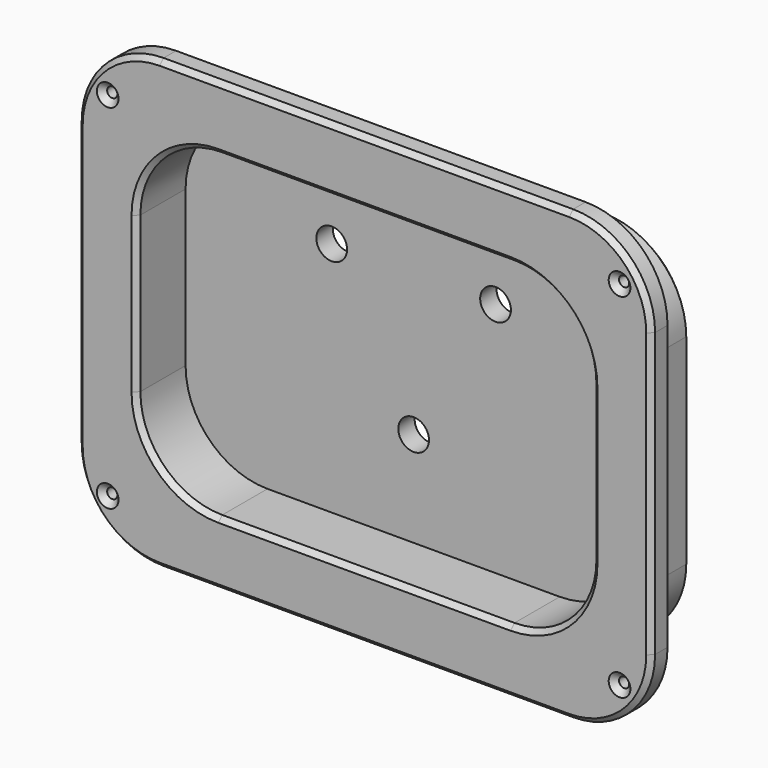
from build123d import *

# Parameters (mm, degrees)
F0_W      = 177.8
F0_H      = 138.684
F1_DEPTH  = 25.4
F2_W      = 177.8
F2_H      = 138.684
F2_W_2    = 161.3722443581
F2_H_2    = 112.8829941154
F3_DEPTH  = 19.05
F4_W      = 141.4277553558
F4_H      = 98.9994257689
F5_DEPTH  = 19.05
F6_R      = 25.4
F7_R      = 4.7625
F8_DEPTH  = 6.351
F9_SIZE   = 1.524
F10_R     = 1.5875
F11_DEPTH = 6.351
F12_SIZE  = 1.778


with BuildPart() as f1:
    # F0 (on Front) → F1 (new body)
    with BuildSketch(Plane.XZ):
        Rectangle(F0_W, F0_H)
    extrude(amount=F1_DEPTH)

    # F2 (on face) → F3 (cut)
    with BuildSketch(Plane(origin=(0, 0, 0), x_dir=(-1, 0, 0), z_dir=(0, 1, 0))):
        Rectangle(F2_W, F2_H)
        Rectangle(F2_W_2, F2_H_2, mode=Mode.SUBTRACT)
    extrude(amount=-F3_DEPTH, mode=Mode.SUBTRACT)

    # F4 (on face) → F5 (cut)
    with BuildSketch(Plane.XZ.offset(25.4)):
        Rectangle(F4_W, F4_H)
    extrude(amount=-F5_DEPTH, mode=Mode.SUBTRACT)

    # F6
    f6_edges = [f1.edges().sort_by_distance(p)[0] for p in [
        (88.9, -22.225, 69.342),
        (88.9, -22.225, -69.342),
        (-88.9, -22.225, -69.342),
        (-88.9, -22.225, 69.342),
        (-70.713878, -15.875, 49.499713),
        (70.713878, -15.875, 49.499713),
        (70.713878, -15.875, -49.499713),
        (-70.713878, -15.875, -49.499713),
        (80.686122, -9.525, -56.441497),
        (80.686122, -9.525, 56.441497),
        (-80.686122, -9.525, -56.441497),
        (-80.686122, -9.525, 56.441497),
    ]]
    fillet(f6_edges, radius=F6_R)

    # F7 (on face) → F8 (cut, through all)
    with BuildSketch(Plane.XZ.offset(6.35)):
        with Locations((-25.4, 23.863709036)):
            Circle(F7_R)
        with Locations((25.4, 23.863709036)):
            Circle(F7_R)
        with Locations((0, -19.9294611812)):
            Circle(F7_R)
    extrude(amount=-F8_DEPTH, mode=Mode.SUBTRACT)

    # F9
    f9_edges = [f1.edges().sort_by_distance(p)[0] for p in [
        (0, -25.4, -49.499713),
        (70.713878, -25.4, 0),
        (-88.9, -25.4, 0),
        (-81.460512, -25.4, -61.902512),
        (0, 0, -56.441497),
        (88.9, -25.4, 0),
        (81.460512, -25.4, 61.902512),
        (81.460512, -25.4, -61.902512),
        (0, -25.4, -69.342),
        (0, -25.4, 69.342),
        (-81.460512, -25.4, 61.902512),
        (-63.27439, -25.4, -42.060225),
        (63.27439, -25.4, -42.060225),
        (-70.713878, -25.4, 0),
        (-63.27439, -25.4, 42.060225),
        (63.27439, -25.4, 42.060225),
        (0, -25.4, 49.499713),
        (-80.686122, 0, 0),
        (-73.246634, 0, 49.002009),
        (-73.246634, 0, -49.002009),
        (0, 0, 56.441497),
        (73.246634, 0, 49.002009),
        (73.246634, 0, -49.002009),
        (80.686122, 0, 0),
    ]]
    chamfer(f9_edges, length=F9_SIZE)

    # F10 (on face) → F11 (cut, through all)
    with BuildSketch(Plane(origin=(0, -19.05, 0), x_dir=(-1, 0, 0), z_dir=(0, 1, 0))):
        with Locations((-79.0948867798, 54.6215597034)):
            Circle(F10_R)
        with Locations((79.6314403415, 54.6215597034)):
            Circle(F10_R)
        with Locations((79.6314403415, -54.8539970577)):
            Circle(F10_R)
        with Locations((-79.0948867798, -54.8539970577)):
            Circle(F10_R)
    extrude(amount=-F11_DEPTH, mode=Mode.SUBTRACT)

    # F12
    f12_edges = [f1.edges().sort_by_distance(p)[0] for p in [
        (-78.04394, -25.4, 54.62156),
        (80.682387, -25.4, 54.62156),
        (80.682387, -25.4, -54.853997),
        (-78.04394, -25.4, -54.853997),
    ]]
    chamfer(f12_edges, length=F12_SIZE)


solid = f1.part
